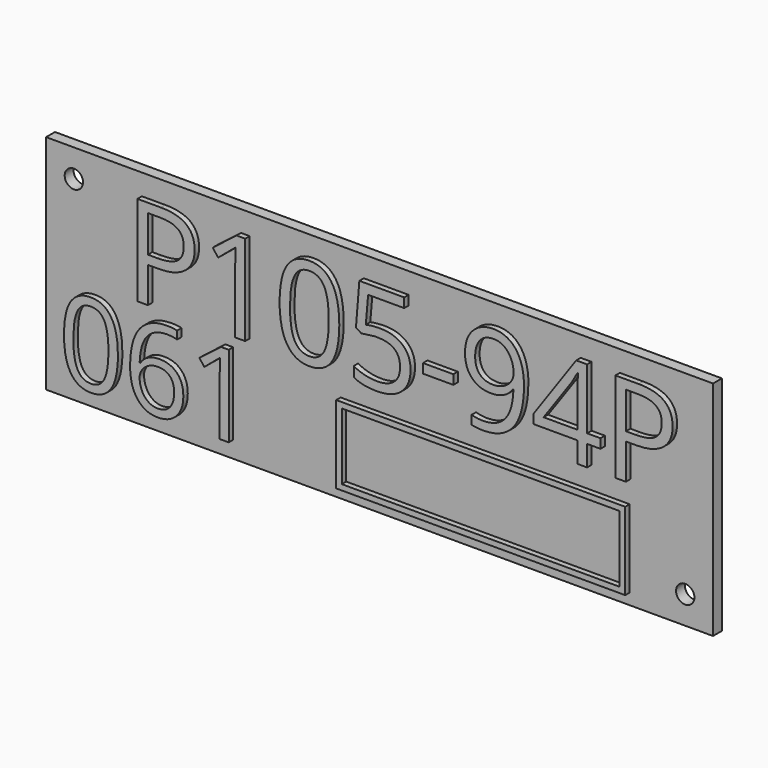
from build123d import *

# Parameters (mm, degrees)
F0_W         = 120
F0_H         = 40
F1_DEPTH     = 2
F3_D         = 3.3
F4_TEXT_SIZE = 22.7377695669
F5_DEPTH     = 1
F6_TEXT_SIZE = 20.5478077656
F7_DEPTH     = 1
F8_W         = 52
F8_H         = 14
F8_W_2       = 49.99999962
F8_H_2       = 11.99999962
F9_DEPTH     = 1


# Not quite as in the source:
# - Text() gives the source's letters only with a copy of the font that has no kerning and outlines rounded to 1/6400 em; it was checked with that copy


with BuildPart() as f1:
    # F0 (on Front) → F1 (new body)
    with BuildSketch(Plane.XZ):
        Rectangle(F0_W, F0_H)
    extrude(amount=F1_DEPTH)

    # F3 (through all)
    with Locations(Plane.XZ.offset(2)):
        with Locations((-55, 15), (55, -15)):
            Hole(F3_D / 2)

    # F4 (on face) → F5 (join)
    with BuildSketch(Plane.XZ.offset(2)):
        with Locations((-45, 0)):
            Text('P105-94P', F4_TEXT_SIZE, font='Open Sans', text_align=(TextAlign.LEFT, TextAlign.BOTTOM))
    extrude(amount=F5_DEPTH)

    # F6 (on face) → F7 (join)
    with BuildSketch(Plane.XZ.offset(2)):
        with Locations((-57, -17)):
            Text('061', F6_TEXT_SIZE, font='Open Sans', text_align=(TextAlign.LEFT, TextAlign.BOTTOM))
    extrude(amount=F7_DEPTH)

    # F8 (on face) → F9 (join)
    with BuildSketch(Plane.XZ.offset(2)):
        with Locations((19, -11)):
            Rectangle(F8_W, F8_H)
        with Locations((19, -11)):
            Rectangle(F8_W_2, F8_H_2, mode=Mode.SUBTRACT)
    extrude(amount=F9_DEPTH)


solid = f1.part
